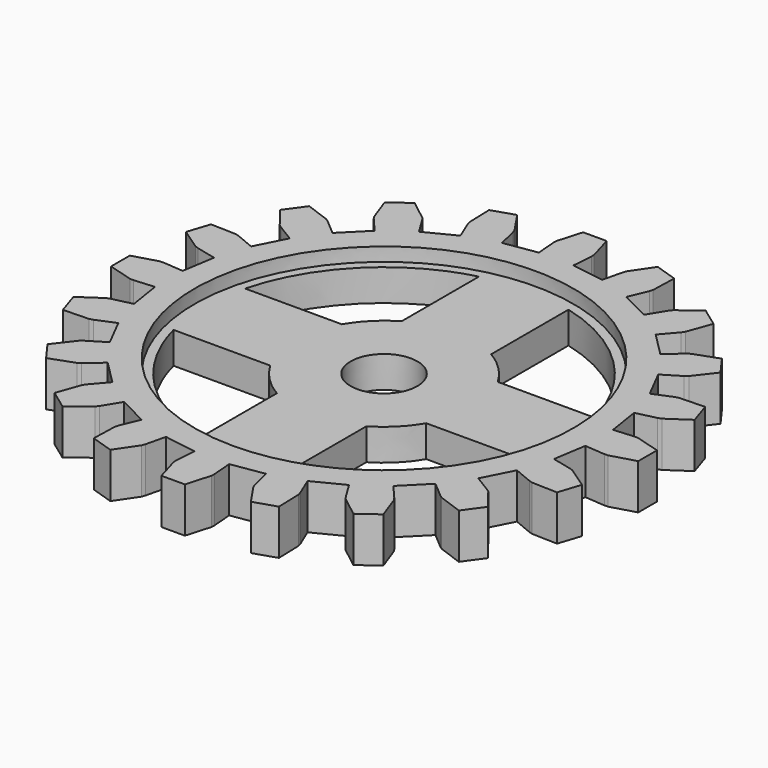
from build123d import *

# Parameters (mm, degrees)
F1_DEPTH = 10
F3_DEPTH = 3
F5_DEPTH = 7


# Not quite as in the source:
# - ends of sketch curves that miss each other by under 0.0002 mm in the source are joined


with BuildPart() as f1:
    # F0 (on Top) → F1 (new body)
    with BuildSketch(Plane.XY):
        Polygon((2.592916, 58.358259), (-2.601737, 58.358259), (-4.171604, 52.94312), (-4.198076, 52.131731), (-3.836479, 47.642634), (-11.077243, 46.496106), (-12.117937, 50.879367), (-12.40016, 51.637839), (-15.56634, 56.303326), (-20.505229, 54.69819), (-20.32884, 49.062565), (-20.108354, 48.286453), (-18.370921, 44.123676), (-24.906132, 40.798742), (-27.252104, 44.644023), (-27.754812, 45.279023), (-32.208626, 48.736242), (-36.406686, 45.684717), (-34.492865, 40.384228), (-34.043073, 39.705134), (-31.106201, 36.292009), (-36.292032, 31.106173), (-39.713979, 34.034231), (-40.384254, 34.492842), (-45.69356, 36.406662), (-48.745089, 32.199787), (-45.287866, 27.745967), (-44.644046, 27.243259), (-40.798769, 24.897284), (-44.123699, 18.370898), (-48.286476, 20.099509), (-49.071408, 20.319995), (-54.707033, 20.505203), (-56.312171, 15.566312), (-51.64668, 12.400134), (-50.879387, 12.117912), (-46.496126, 11.077217), (-47.642654, 3.836453), (-52.131751, 4.198051), (-52.943138, 4.16277), (-58.358277, 2.592909), (-58.358277, -2.592922), (-52.943138, -4.162783), (-52.131751, -4.198063), (-47.642654, -3.836463), (-46.496126, -11.077227), (-50.879387, -12.117922), (-51.64668, -12.400144), (-56.312165, -15.566324), (-54.707028, -20.505216), (-49.071403, -20.320005), (-48.286471, -20.099522), (-44.123693, -18.370911), (-40.798763, -24.897297), (-44.64404, -27.243269), (-45.287861, -27.745977), (-48.745084, -32.199797), (-45.693554, -36.406674), (-40.384249, -34.492852), (-39.713973, -34.034241), (-36.292027, -31.106185), (-31.106196, -36.292019), (-34.043068, -39.705147), (-34.492859, -40.384241), (-36.406681, -45.684713), (-32.20862, -48.73623), (-27.754807, -45.279019), (-27.252098, -44.644033), (-24.906126, -40.798755), (-18.370915, -44.123688), (-20.108348, -48.277618), (-20.328834, -49.062535), (-20.505223, -54.698174), (-15.566334, -56.303313), (-12.400154, -51.637813), (-12.117932, -50.879369), (-11.077237, -46.496102), (-3.836473, -47.64263), (-4.198071, -52.131702), (-4.171598, -52.94309), (-2.601737, -58.358258), (2.592916, -58.358258), (4.162777, -52.94309), (4.189249, -52.131702), (3.827652, -47.64263), (11.068416, -46.496102), (12.11793, -50.879369), (12.391333, -51.637813), (15.557513, -56.303313), (20.496402, -54.698174), (20.320013, -49.062535), (20.099527, -48.277618), (18.362097, -44.123688), (24.897305, -40.798755), (27.243277, -44.644033), (27.745985, -45.279019), (32.199805, -48.73623), (36.39786, -45.684713), (34.484041, -40.384241), (34.034249, -39.705147), (31.106194, -36.292019), (36.283208, -31.106185), (39.705152, -34.034241), (40.37543, -34.492852), (45.684735, -36.406674), (48.736263, -32.199797), (45.279041, -27.745977), (44.635222, -27.243269), (40.789944, -24.897297), (44.123694, -18.370911), (48.277652, -20.099522), (49.062583, -20.320005), (54.698208, -20.505216), (56.303344, -15.566324), (51.63786, -12.400144), (50.870569, -12.117922), (46.487305, -11.077227), (47.633833, -3.836463), (52.12293, -4.198063), (52.943138, -4.162783), (58.358277, -2.592922), (58.358277, 2.592909), (52.943138, 4.16277), (52.12293, 4.198051), (47.633833, 3.836453), (46.487305, 11.077217), (50.870569, 12.117912), (51.63786, 12.400134), (56.303344, 15.566312), (54.698208, 20.505203), (49.062583, 20.319995), (48.277652, 20.099509), (44.123694, 18.370898), (40.789944, 24.897284), (44.635222, 27.243259), (45.279041, 27.745967), (48.736263, 32.199787), (45.684735, 36.406662), (40.37543, 34.492842), (39.705152, 34.034231), (36.283208, 31.106173), (31.106194, 36.292009), (34.034249, 39.705134), (34.484041, 40.384228), (36.39786, 45.684717), (32.199805, 48.736242), (27.745985, 45.279023), (27.243277, 44.644023), (24.897305, 40.798742), (18.362097, 44.123676), (20.099527, 48.286453), (20.320013, 49.062565), (20.496402, 54.69819), (15.557513, 56.303326), (12.391333, 51.637839), (12.11793, 50.879367), (11.068416, 46.496106), (3.827652, 47.642634), (4.189249, 52.131731), (4.162777, 52.94312), align=None)
    extrude(amount=F1_DEPTH)

    # F2 (on face) → F3 (cut)
    with BuildSketch(Plane.XY.offset(10)):
        with BuildLine():
            add(Edge.make_bspline(
                [(41.899994, -1.3e-05), (41.899994, -23.140745), (23.140726, -41.900014), (-4e-06, -41.900014)],
                knots=[0, 0, 0, 0, 1, 1, 1, 1], degree=3))
            add(Edge.make_bspline(
                [(-4e-06, 41.899987), (23.140726, 41.899987), (41.899994, 23.140716), (41.899994, -1.3e-05)],
                knots=[0, 0, 0, 0, 1, 1, 1, 1], degree=3))
            add(Edge.make_bspline(
                [(-41.900003, -1.3e-05), (-41.900003, 23.140716), (-23.140736, 41.899987), (-4e-06, 41.899987)],
                knots=[0, 0, 0, 0, 1, 1, 1, 1], degree=3))
            add(Edge.make_bspline(
                [(-4e-06, -41.900014), (-23.140736, -41.900014), (-41.900003, -23.140745), (-41.900003, -1.3e-05)],
                knots=[0, 0, 0, 0, 1, 1, 1, 1], degree=3))
        make_face()
    extrude(amount=-F3_DEPTH, mode=Mode.SUBTRACT)

    # F4 (on face) → F5 (cut, through all)
    with BuildSketch(Plane.XY.offset(7)):
        with BuildLine():
            add(Edge.make_bspline(
                [(-9.904243, 17.259648), (-12.960057, 15.502507), (-15.502521, 12.960046), (-17.259659, 9.904231)],
                knots=[0, 0, 0, 0, 1, 1, 1, 1], degree=3))
            Line((-9.904243, 17.259648), (-9.904243, 38.664437))
            add(Edge.make_bspline(
                [(-38.67327, 9.904231), (-35.076585, 23.984642), (-23.986248, 35.069349), (-9.904243, 38.664437)],
                knots=[0, 0, 0, 0, 1, 1, 1, 1], degree=3))
            Line((-38.67327, 9.904231), (-17.259659, 9.904231))
        make_face()
        with BuildLine():
            add(Edge.make_bspline(
                [(9.90423, 38.664437), (23.984641, 35.069349), (35.069347, 23.984642), (38.664438, 9.904231)],
                knots=[0, 0, 0, 0, 1, 1, 1, 1], degree=3))
            Line((9.90423, 38.664437), (9.90423, 17.259648))
            add(Edge.make_bspline(
                [(17.259646, 9.904231), (15.502508, 12.960046), (12.960044, 15.502507), (9.90423, 17.259648)],
                knots=[0, 0, 0, 0, 1, 1, 1, 1], degree=3))
            Line((17.259646, 9.904231), (38.664438, 9.904231))
        make_face()
        with BuildLine():
            add(Edge.make_bspline(
                [(-7e-06, 7.399509), (4.086901, 7.399509), (7.399507, 4.086903), (7.399507, -5e-06)],
                knots=[0, 0, 0, 0, 1, 1, 1, 1], degree=3))
            add(Edge.make_bspline(
                [(-7.39952, -5e-06), (-7.39952, 4.086903), (-4.086914, 7.399509), (-7e-06, 7.399509)],
                knots=[0, 0, 0, 0, 1, 1, 1, 1], degree=3))
            add(Edge.make_bspline(
                [(-7e-06, -7.399519), (-4.086914, -7.399519), (-7.39952, -4.086916), (-7.39952, -5e-06)],
                knots=[0, 0, 0, 0, 1, 1, 1, 1], degree=3))
            add(Edge.make_bspline(
                [(7.399507, -5e-06), (7.399507, -4.086916), (4.086901, -7.399519), (-7e-06, -7.399519)],
                knots=[0, 0, 0, 0, 1, 1, 1, 1], degree=3))
        make_face()
        with BuildLine():
            add(Edge.make_bspline(
                [(-17.259659, -9.904241), (-15.502521, -12.960056), (-12.960057, -15.50252), (-9.904243, -17.259658)],
                knots=[0, 0, 0, 0, 1, 1, 1, 1], degree=3))
            Line((-17.259659, -9.904241), (-38.67327, -9.904241))
            add(Edge.make_bspline(
                [(-9.904243, -38.664449), (-23.986248, -35.069362), (-35.076585, -23.984652), (-38.67327, -9.904241)],
                knots=[0, 0, 0, 0, 1, 1, 1, 1], degree=3))
            Line((-9.904243, -38.664449), (-9.904243, -17.259658))
        make_face()
        with BuildLine():
            add(Edge.make_bspline(
                [(38.664438, -9.904241), (35.069347, -23.984652), (23.984641, -35.069362), (9.90423, -38.664449)],
                knots=[0, 0, 0, 0, 1, 1, 1, 1], degree=3))
            Line((38.664438, -9.904241), (17.259646, -9.904241))
            add(Edge.make_bspline(
                [(9.90423, -17.259658), (12.960044, -15.50252), (15.502508, -12.960056), (17.259646, -9.904241)],
                knots=[0, 0, 0, 0, 1, 1, 1, 1], degree=3))
            Line((9.90423, -17.259658), (9.90423, -38.664449))
        make_face()
    extrude(amount=-F5_DEPTH, mode=Mode.SUBTRACT)


solid = f1.part
